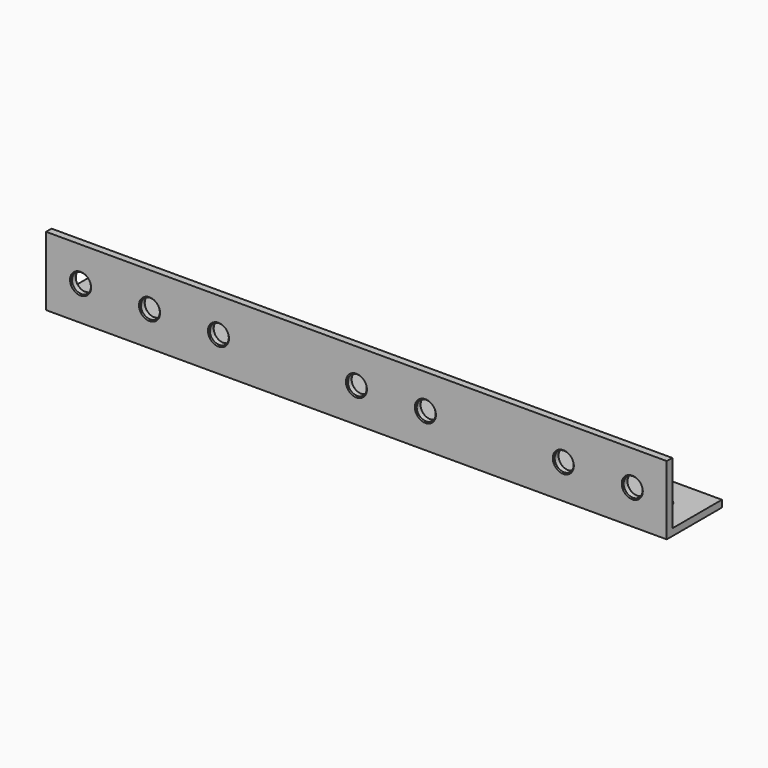
from build123d import *

# Parameters (mm, degrees)
F1_DEPTH = 180
F2_R     = 2.75
F3_DEPTH = 2.001
F4_R     = 2.75
F5_DEPTH = 20.001
F6_SIZE  = 0.3


# Not quite as in the source:
# - a feature names something its author has since deleted; it is built from what else it names


with BuildPart() as f1:
    # F0 (on Right) → F1 (new body)
    with BuildSketch(Plane.YZ):
        Polygon((0, 20), (0, 0), (20, 0), (20, 2), (2, 2), (2, 20), align=None)
    extrude(amount=-F1_DEPTH)

    # F2 (on face) → F3 (cut, through all)
    with BuildSketch(Plane.XY.offset(2)):
        with Locations((-10, 10)):
            Circle(F2_R)
        with Locations((-170, 10)):
            Circle(F2_R)
        with Locations((-150, 10)):
            Circle(F2_R)
        with Locations((-90, 10)):
            Circle(F2_R)
        with Locations((-70, 10)):
            Circle(F2_R)
        with Locations((-30, 10)):
            Circle(F2_R)
        with Locations((-130, 10)):
            Circle(F2_R)
    extrude(amount=-F3_DEPTH, mode=Mode.SUBTRACT)

    # F4 (on face) → F5 (cut, through all)
    with BuildSketch(Plane.XZ):
        with Locations((-170, 10)):
            Circle(F4_R)
        with Locations((-150, 10)):
            Circle(F4_R)
        with Locations((-90, 10)):
            Circle(F4_R)
        with Locations((-70, 10)):
            Circle(F4_R)
        with Locations((-30, 10)):
            Circle(F4_R)
        with Locations((-10, 10)):
            Circle(F4_R)
        with Locations((-130, 10)):
            Circle(F4_R)
    extrude(amount=-F5_DEPTH, mode=Mode.SUBTRACT)

    # F6
    f6_edges = [f1.edges().sort_by_distance(p)[0] for p in [
        (-172.75, 10, 2),
        (-167.25, 10, 1),
        (-172.75, 10, 0),
        (-152.75, 10, 2),
        (-147.25, 10, 1),
        (-152.75, 10, 0),
        (-92.75, 10, 2),
        (-87.25, 10, 1),
        (-92.75, 10, 0),
        (-72.75, 10, 2),
        (-67.25, 10, 1),
        (-72.75, 10, 0),
        (-32.75, 10, 2),
        (-27.25, 10, 1),
        (-32.75, 10, 0),
        (-12.75, 10, 2),
        (-7.25, 10, 1),
        (-12.75, 10, 0),
        (-12.75, 0, 10),
        (-7.25, 1, 10),
        (-12.75, 2, 10),
        (-32.75, 0, 10),
        (-27.25, 1, 10),
        (-32.75, 2, 10),
        (-72.75, 0, 10),
        (-67.25, 1, 10),
        (-72.75, 2, 10),
        (-92.75, 0, 10),
        (-87.25, 1, 10),
        (-92.75, 2, 10),
        (-152.75, 0, 10),
        (-147.25, 1, 10),
        (-152.75, 2, 10),
        (-172.75, 0, 10),
        (-167.25, 1, 10),
        (-172.75, 2, 10),
        (-132.75, 10, 0),
        (-132.75, 10, 2),
        (-132.75, 0, 10),
        (-127.25, 1, 10),
        (-132.75, 2, 10),
    ]]
    chamfer(f6_edges, length=F6_SIZE)


solid = f1.part
